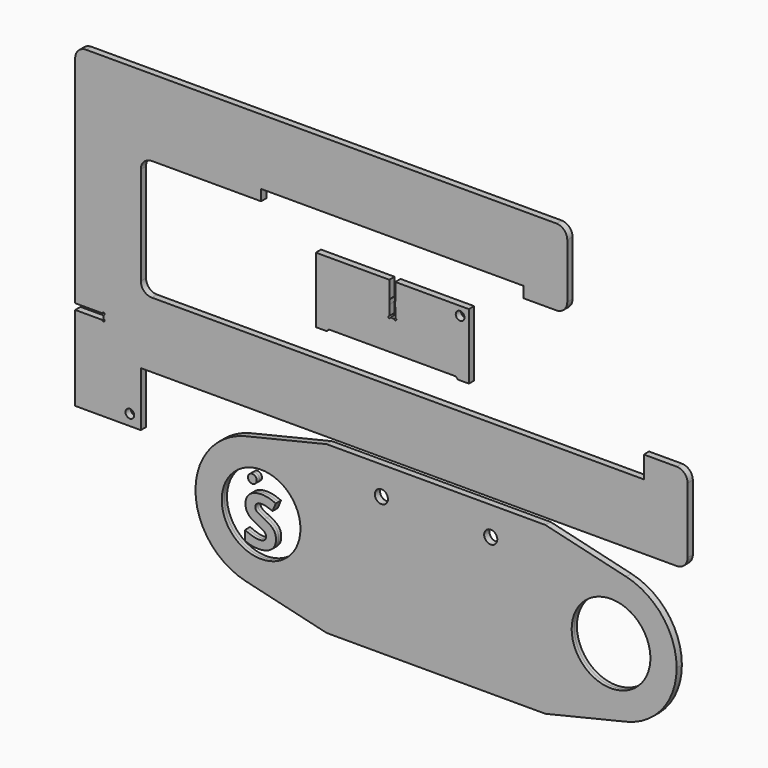
from build123d import *

# Parameters (mm, degrees)
F0_R         = 2
F1_DEPTH     = 1.5
F2_R         = 3
F3_DEPTH     = 1.5
F4_TEXT_SIZE = 30.5555555556
F5_DEPTH     = 1.5
F4_R         = 2
F6_DEPTH     = 1.5
F8_DEPTH     = 12.5
F9_R         = 2
F10_DEPTH    = 1.5
F11_R        = 5


# Not quite as in the source:
# - Text() gives the source's letters only with a copy of the font that has no kerning and outlines rounded to 1/6400 em; it was checked with that copy


with BuildPart() as f1:
    # F0 (on Front) → F1 (new body, symmetric)
    with BuildSketch(Plane.XZ):
        Polygon((60, 32.5), (60, 27.5), (80, 27.5), (80, 62.5), (-145, 62.5), (-145, -57.5), (-145, -82.5), (-115, -82.5), (-115, -57.5), (135, -57.5), (135, -17.5), (115, -17.5), (115, -27.5), (-115, -27.5), (-115, 27.5), (-60, 27.5), (-60, 32.5), align=None)
        with Locations((-120, -77.5)):
            Circle(F0_R, mode=Mode.SUBTRACT)
    extrude(amount=F1_DEPTH, both=True)

    # F7 (on Front) → F8 (cut, symmetric)
    with BuildSketch(Plane.XZ):
        with BuildLine():
            Line((-145, -41.15), (-145, -42.5))
            Line((-145, -42.5), (-145, -43.85))
            Line((-145, -43.85), (-132.5, -43.85))
            ThreePointArc((-132.5, -43.85), (-131.6464466094, -44.2035533906), (-132, -43.35))
            Line((-132, -43.35), (-132, -42.5))
            Line((-132, -42.5), (-132, -41.65))
            ThreePointArc((-132, -41.65), (-131.6464466094, -40.7964466094), (-132.5, -41.15))
            Line((-132.5, -41.15), (-145, -41.15))
        make_face()
    extrude(amount=F8_DEPTH, both=True, mode=Mode.SUBTRACT)

    # F11
    f11_edges = [f1.edges().sort_by_distance(p)[0] for p in [
        (-145, 0, 62.5),
        (80, 0, 62.5),
        (80, 0, 27.5),
        (135, 0, -17.5),
        (135, 0, -57.5),
        (-115, 0, -27.5),
        (-115, 0, 27.5),
    ]]
    fillet(f11_edges, radius=F11_R)


with BuildPart() as f3:
    # F2 (on Front) → F3 (new body, symmetric)
    with BuildSketch(Plane.XZ):
        with BuildLine():
            Line((-30, -60.5), (-66.9624573379, -69.319112628))
            ThreePointArc((-66.9624573379, -69.319112628), (-83.546482966, -79.9106713426), (-90, -98.5))
            ThreePointArc((-90, -98.5), (-83.546482966, -117.0893286574), (-66.9624573379, -127.680887372))
            Line((-66.9624573379, -127.680887372), (-30, -136.5))
            Line((-30, -136.5), (20, -136.5))
            Line((20, -136.5), (70, -136.5))
            Line((70, -136.5), (106.9624573379, -127.680887372))
            ThreePointArc((106.9624573379, -127.680887372), (123.546482966, -117.0893286574), (130, -98.5))
            ThreePointArc((130, -98.5), (123.546482966, -79.9106713426), (106.9624573379, -69.319112628))
            Line((106.9624573379, -69.319112628), (70, -60.5))
            Line((70, -60.5), (20, -60.5))
            Line((20, -60.5), (-30, -60.5))
        make_face()
        with BuildLine():
            ThreePointArc((-78, -98.5), (-60, -80.5), (-42, -98.5))
            ThreePointArc((-42, -98.5), (-60, -116.5), (-78, -98.5))
        make_face(mode=Mode.SUBTRACT)
        with Locations((-5, -73.5)):
            Circle(F2_R, mode=Mode.SUBTRACT)
        with BuildLine():
            ThreePointArc((118, -98.5), (100, -116.5), (82, -98.5))
            ThreePointArc((82, -98.5), (100, -80.5), (118, -98.5))
        make_face(mode=Mode.SUBTRACT)
        with Locations((45, -73.5)):
            Circle(F2_R, mode=Mode.SUBTRACT)
    extrude(amount=F3_DEPTH, both=True)


with BuildPart() as f5:
    # F4 (on Front) → F5 (new body, symmetric)
    with BuildSketch(Plane.XZ):
        with Locations((-68.8014322917, -112.5)):
            Text('S', F4_TEXT_SIZE, font='Open Sans', font_style=FontStyle.BOLD, text_align=(TextAlign.LEFT, TextAlign.BOTTOM))
    extrude(amount=F5_DEPTH, both=True)

    # F4 (on Front) → F6 (join, symmetric)
    with BuildSketch(Plane.XZ):
        with Locations((-64, -85.5)):
            Circle(F4_R)
        with Locations((-68.8014322917, -112.5)):
            Text('S', F4_TEXT_SIZE, font='Open Sans', font_style=FontStyle.BOLD, text_align=(TextAlign.LEFT, TextAlign.BOTTOM))
    extrude(amount=F6_DEPTH, both=True)


with BuildPart() as f10:
    # F9 (on Front) → F10 (new body, symmetric)
    with BuildSketch(Plane.XZ):
        with BuildLine():
            Line((-35, 15), (-35, -15))
            Line((-35, -15), (-30, -15))
            Line((-30, -15), (-29, -14))
            Line((-29, -14), (0, -14))
            Line((0, -14), (29, -14))
            Line((29, -14), (30, -15))
            Line((30, -15), (35, -15))
            Line((35, -15), (35, 15))
            Line((35, 15), (1.35, 15))
            Line((1.35, 15), (1.35, 7.2))
            Line((1.35, 7.2), (1.25, 7.1))
            Line((1.25, 7.1), (1.25, 5.1))
            Line((1.25, 5.1), (1.35, 5))
            Line((1.35, 5), (1.35, 0.5))
            ThreePointArc((1.35, 0.5), (1.7035533906, -0.3535533906), (0.85, 0))
            Line((0.85, 0), (0, 0))
            Line((0, 0), (-0.85, 0))
            ThreePointArc((-0.85, 0), (-1.7035533906, -0.3535533906), (-1.35, 0.5))
            Line((-1.35, 0.5), (-1.35, 5))
            Line((-1.35, 5), (-1.25, 5.1))
            Line((-1.25, 5.1), (-1.25, 7.1))
            Line((-1.25, 7.1), (-1.35, 7.2))
            Line((-1.35, 7.2), (-1.35, 15))
            Line((-1.35, 15), (-35, 15))
        make_face()
        with Locations((31, 11)):
            Circle(F9_R, mode=Mode.SUBTRACT)
    extrude(amount=F10_DEPTH, both=True)


solid = Compound([f1.part, f3.part, f5.part, f10.part])
